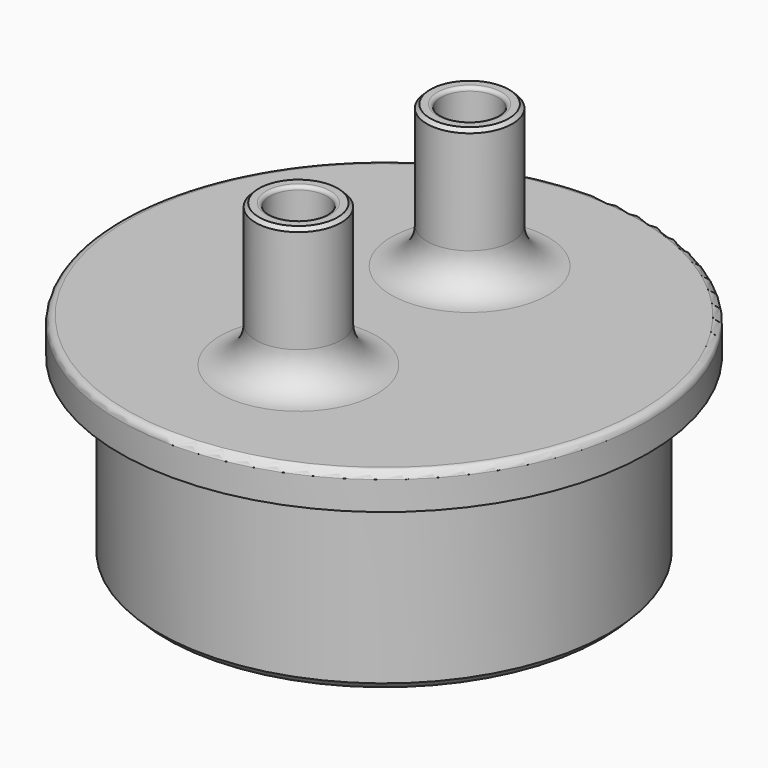
from build123d import *

# Parameters (mm, degrees)
F0_R     = 31.5
F0_R_2   = 26.5
F1_DEPTH = 25
F2_R     = 37
F2_R_2   = 31.5
F2_R_3   = 26.5
F3_DEPTH = 5
F4_R     = 6
F4_R_2   = 4
F5_DEPTH = 20
F7_R     = 1
F8_SIZE  = 1
F9_R     = 0.5
F10_SIZE = 0.5
F11_SIZE = 0.5
F12_SIZE = 0.5


# Not quite as in the source:
# - a fillet or chamfer that OpenCascade refuses, or shapes differently, is made with other operations: its cross-section is extruded or revolved along the edge and cut away or added


with BuildPart() as f1:
    # F0 (on Top) → F1 (new body)
    with BuildSketch(Plane.XY):
        Circle(F0_R)
        Circle(F0_R_2, mode=Mode.SUBTRACT)
    extrude(amount=F1_DEPTH)

    # F2 (on face) → F3 (join)
    with BuildSketch(Plane.XY.offset(25)):
        Circle(F2_R)
        Circle(F2_R_2, mode=Mode.SUBTRACT)
        Circle(F2_R_2)
        Circle(F2_R_3, mode=Mode.SUBTRACT)
        Circle(F2_R_3)
    extrude(amount=F3_DEPTH)

    # F4 (on face) → F5 (join, symmetric)
    with BuildSketch(Plane.XY.offset(30)):
        with Locations((0, -15)):
            Circle(F4_R)
        with Locations((0, -15)):
            Circle(F4_R_2, mode=Mode.SUBTRACT)
        with Locations((0, 15)):
            Circle(F4_R)
        with Locations((0, 15)):
            Circle(F4_R_2, mode=Mode.SUBTRACT)
    extrude(amount=F5_DEPTH, both=True)

    # F6: fillet of radius 5 on 5 edges, made by hand

    # F6_s1 → F6_t2 (revolve)
    with BuildSketch(Plane.XZ.offset(-15)):
        with BuildLine():
            ThreePointArc((11, 30), (7.4644660941, 31.4644660941), (6, 35))
            Line((6, 35), (6, 30))
            Line((6, 30), (11, 30))
        make_face()
    revolve(axis=Axis((0, 15, 30), (0, 0, 1)))

    # F6_s3 → F6_t4 (revolve)
    with BuildSketch(Plane.XZ.offset(15)):
        with BuildLine():
            ThreePointArc((11, 30), (7.4644660941, 31.4644660941), (6, 35))
            Line((6, 35), (6, 30))
            Line((6, 30), (11, 30))
        make_face()
    revolve(axis=Axis((0, -15, 30), (0, 0, 1)))

    # F6_s5 → F6_t6 (revolve)
    with BuildSketch(Plane.XZ):
        with BuildLine():
            ThreePointArc((26.5, 20), (25.0355339059, 23.5355339059), (21.5, 25))
            Line((21.5, 25), (26.5, 25))
            Line((26.5, 25), (26.5, 20))
        make_face()
    revolve(axis=Axis((0, 0, 25), (0, 0, 1)))

    # F6_s7 → F6_t8 (revolve)
    with BuildSketch(Plane.XZ.offset(15)):
        with BuildLine():
            ThreePointArc((11, 25), (7.4644660941, 23.5355339059), (6, 20))
            Line((6, 20), (6, 25))
            Line((6, 25), (11, 25))
        make_face()
    revolve(axis=Axis((0, -15, 25), (0, 0, 1)))

    # F6_s9 → F6_t10 (revolve)
    with BuildSketch(Plane.XZ.offset(-15)):
        with BuildLine():
            ThreePointArc((11, 25), (7.4644660941, 23.5355339059), (6, 20))
            Line((6, 20), (6, 25))
            Line((6, 25), (11, 25))
        make_face()
    revolve(axis=Axis((0, 15, 25), (0, 0, 1)))

    # F7
    f7_edges = [f1.edges().sort_by_distance(p)[0] for p in [
        (-37, 0, 30),
    ]]
    fillet(f7_edges, radius=F7_R)

    # F8
    f8_edges = [f1.edges().sort_by_distance(p)[0] for p in [
        (-31.5, 0, 0),
    ]]
    chamfer(f8_edges, length=F8_SIZE)

    # F9
    f9_edges = [f1.edges().sort_by_distance(p)[0] for p in [
        (4, 15, 40),
        (-4, 15, 30),
        (-4, 15, 50),
        (4, -15, 40),
        (-4, -15, 30),
        (-4, -15, 50),
    ]]
    fillet(f9_edges, radius=F9_R)

    # F10
    f10_edges = [f1.edges().sort_by_distance(p)[0] for p in [
        (-6, -15, 50),
        (-6, 15, 50),
    ]]
    chamfer(f10_edges, length=F10_SIZE)

    # F11
    f11_edges = [f1.edges().sort_by_distance(p)[0] for p in [
        (-4, 15, 10),
        (-4, -15, 10),
    ]]
    chamfer(f11_edges, length=F11_SIZE)

    # F12
    f12_edges = [f1.edges().sort_by_distance(p)[0] for p in [
        (-6, 15, 10),
        (-6, -15, 10),
    ]]
    chamfer(f12_edges, length=F12_SIZE)


solid = f1.part
